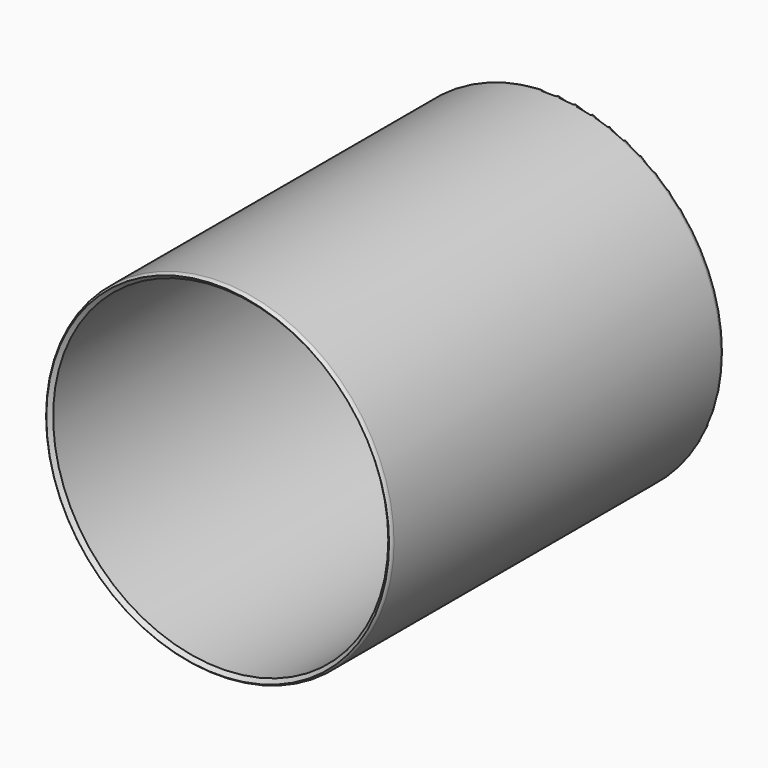
from build123d import *

# Parameters (mm, degrees)
F0_R     = 37.3678316612
F0_R_2   = 36.1312756735
F1_DEPTH = 90
F2_R     = 1


# Not quite as in the source:
# - a fillet or chamfer that OpenCascade refuses, or shapes differently, is made with other operations: its cross-section is extruded or revolved along the edge and cut away or added


with BuildPart() as f1:
    # F0 (on Front) → F1 (new body)
    with BuildSketch(Plane.XZ):
        Circle(F0_R)
        Circle(F0_R_2, mode=Mode.SUBTRACT)
    extrude(amount=F1_DEPTH)

    # F2
    f2_edges = [f1.edges().sort_by_distance(p)[0] for p in [
        (37.367832, -45, 0),
        (-37.367832, 0, 0),
        (-37.367832, -90, 0),
    ]]
    fillet(f2_edges, radius=F2_R)

    # F3: chamfer of 1 on 2 edges, made by hand

    # F3_s1 → F3_t2 (revolve, cut)
    with BuildSketch(Plane.XY):
        Polygon((37.1312756735, -90), (36.1312756735, -89), (36.1312756735, -90), align=None)
    revolve(axis=Axis((0, -90, 0), (0, -1, 0)), mode=Mode.SUBTRACT)


solid = f1.part
